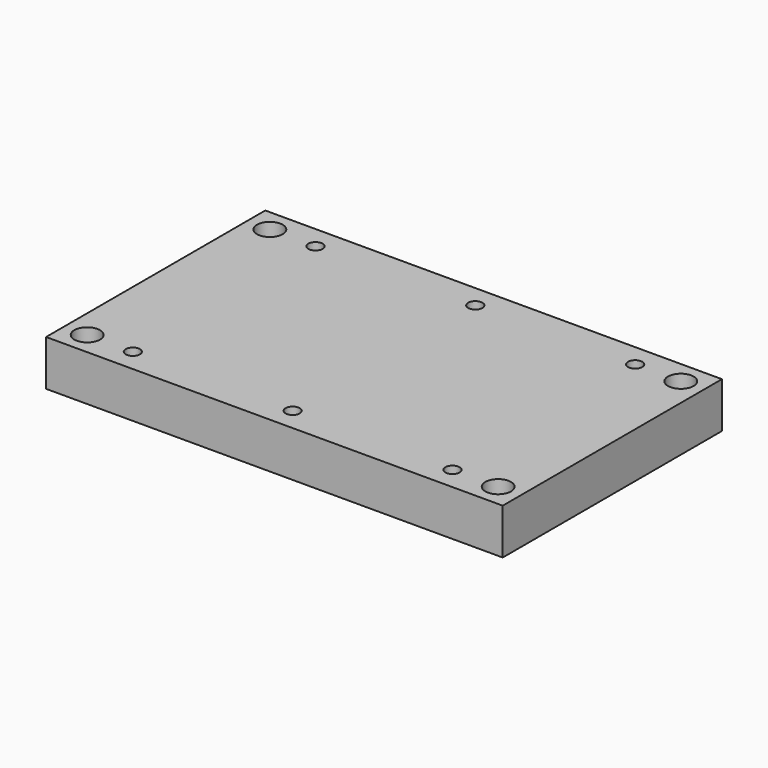
from build123d import *

# Parameters (mm, degrees)
F0_W           = 254
F0_H           = 152.4
F1_DEPTH       = 25.4
F3_D           = 9.525
F3_CBORE_D     = 14.2875
F3_CBORE_DEPTH = 12.7
F5_D           = 7.9375


# Not quite as in the source:
# - a length typed as a fraction of an inch, garbled in the dataset ("3 / 203.2 mm" for 3/8 in), is restored


with BuildPart() as f1:
    # F0 (on Top) → F1 (new body)
    with BuildSketch(Plane.XY):
        Rectangle(F0_W, F0_H)
    extrude(amount=F1_DEPTH)

    # F3 (through all)
    with Locations(Plane.XY.offset(25.4)):
        with Locations((-114.3, 63.5), (-114.3, -63.5), (114.3, 63.5), (114.3, -63.5)):
            CounterBoreHole(F3_D / 2, F3_CBORE_D / 2, F3_CBORE_DEPTH)

    # F5 (through all)
    with Locations(Plane.XY.offset(25.4)):
        with Locations((-88.9, 63.5), (0, 63.5), (88.9, 63.5), (88.9, -63.5), (0, -63.5), (-88.9, -63.5)):
            Hole(F5_D / 2)


solid = f1.part
